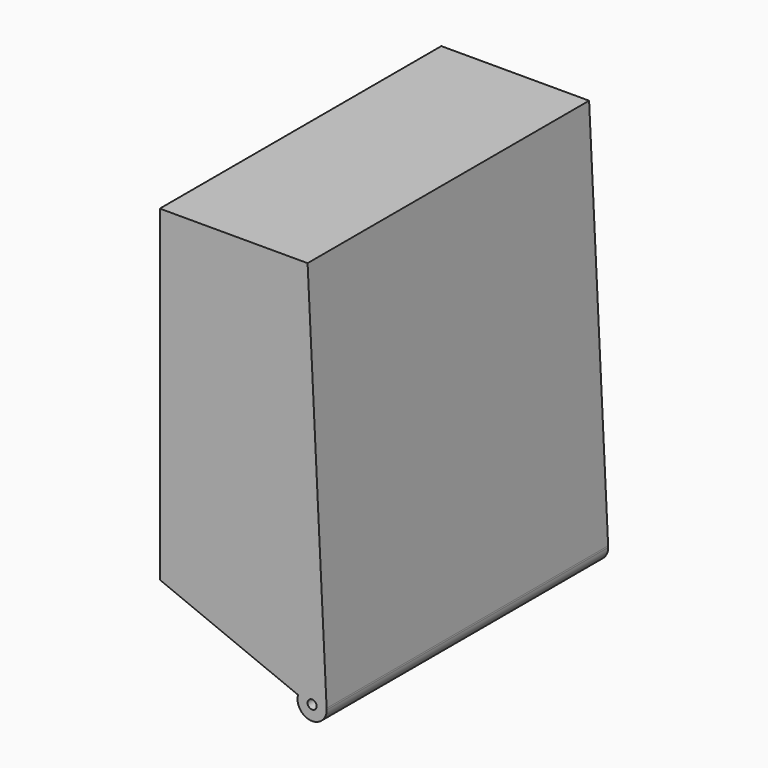
from build123d import *

# Parameters (mm, degrees)
F0_W     = 70
F0_H     = 77
F1_DEPTH = 29.4
F2_W     = 25.4
F2_H     = 66
F3_DEPTH = 75
F5_DEPTH = 70
F6_R     = 0.9
F7_DEPTH = 70
F8_DEPTH = 70


with BuildPart() as f1:
    # F0 (on Right) → F1 (new body)
    with BuildSketch(Plane.YZ):
        with Locations((35, 38.5)):
            Rectangle(F0_W, F0_H)
    extrude(amount=F1_DEPTH)

    # F2 (on Top) → F3 (cut)
    with BuildSketch(Plane.XY):
        with Locations((14.7, 35)):
            Rectangle(F2_W, F2_H)
    extrude(amount=F3_DEPTH, mode=Mode.SUBTRACT)

    # F4 (on face) → F5 (cut, through all)
    with BuildSketch(Plane(origin=(0, 70, 0), x_dir=(-1, 0, 0), z_dir=(0, 1, 0))):
        Polygon((0, 0), (0, 12), (-29.4, 0), align=None)
    extrude(amount=-F5_DEPTH, mode=Mode.SUBTRACT)

    # F6 (on face) → F7 (join)
    with BuildSketch(Plane(origin=(0, 70, 0), x_dir=(-1, 0, 0), z_dir=(0, 1, 0))):
        with BuildLine():
            ThreePointArc((-33.1859084974, 0.2855383414), (-31.8851667844, 2.4284246469), (-29.4, 2.7568097504))
            Line((-29.4, 2.7568097504), (-29.4, 77))
            Line((-29.4, 77), (-33.1859084974, 0.2855383414))
        make_face()
        with BuildLine():
            Line((-27.5050449892, 0.7734510248), (-29.4, 0))
            Line((-29.4, 0), (-29.4, 2.7568097504))
            ThreePointArc((-29.4, 2.7568097504), (-31.8851667844, 2.4284246469), (-33.1859084974, 0.2855383414))
            Line((-33.1859084974, 0.2855383414), (-33.2, 0))
            ThreePointArc((-33.2, 0), (-30.3, -2.9), (-27.4, 0))
            ThreePointArc((-27.4, 0), (-27.4263812421, 0.390275844), (-27.5050449892, 0.7734510248))
        make_face()
        with Locations((-30.3, 0)):
            Circle(F6_R, mode=Mode.SUBTRACT)
        with Locations((-30.3, 0)):
            Circle(F6_R)
    extrude(amount=-F7_DEPTH)

    # F6 (on face) → F8 (cut, through all)
    with BuildSketch(Plane(origin=(0, 70, 0), x_dir=(-1, 0, 0), z_dir=(0, 1, 0))):
        with Locations((-30.3, 0)):
            Circle(F6_R)
    extrude(amount=-F8_DEPTH, mode=Mode.SUBTRACT)


solid = f1.part
